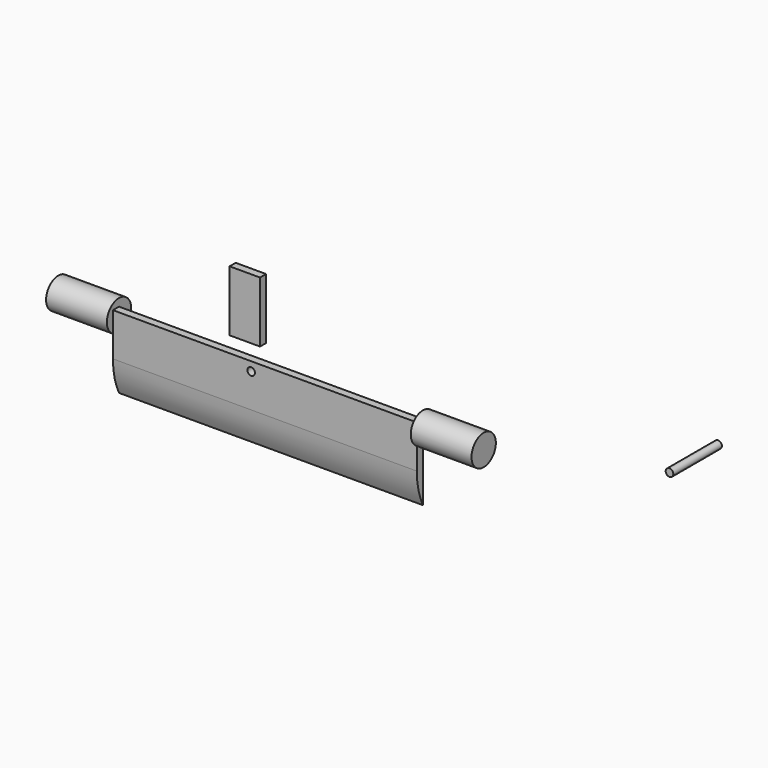
from build123d import *

# Parameters (mm, degrees)
F0_W        = 10.16
F0_H        = 2.54
F3_DEPTH    = 1.27
F4_T1_DEPTH = 78.4790082915
F5_R        = 0.635
F6_DEPTH    = 3.811
F7_DEPTH    = 10.16
F8_DEPTH    = 1.27


# Not quite as in the source:
# - a fillet or chamfer that OpenCascade refuses, or shapes differently, is made with other operations: its cross-section is extruded or revolved along the edge and cut away or added


with BuildPart() as f1:
    # F0 (on Front) → F1 (revolve)
    with BuildSketch(Plane.XZ):
        with Locations((-53.6708150854, 36.4173984443)):
            Rectangle(F0_W, F0_H)
    revolve(axis=Axis((-53.6708150854, 0, 37.6873984443), (-1, 0, 0)))


with BuildPart() as f2:
    # F0 (on Front) → F2 (revolve)
    with BuildSketch(Plane.XZ):
        with Locations((7.2891849146, 36.4173984443)):
            Rectangle(F0_W, F0_H)
    revolve(axis=Axis((7.2891849146, 0, 37.6873984443), (1, 0, 0)))


with BuildPart() as f3:
    # F0 (on Front) → F3 (new body)
    with BuildSketch(Plane.XZ):
        Polygon((-48.5908150854, 26.2573984443), (2.2091849146, 26.2573984443), (2.2091849146, 35.1473984443), (2.2091849146, 37.6873984443), (2.2091849146, 38.9573984443), (-48.5908150854, 38.9573984443), (-48.5908150854, 37.6873984443), (-48.5908150854, 35.1473984443), align=None)
    extrude(amount=F3_DEPTH)

    # F4: fillet of radius 12.7 on 1 edges, made by hand

    # F4_s2 → F4_t1 (cut)
    with BuildSketch(Plane.YZ.offset(-62.4303192311)):
        with BuildLine():
            add(Edge.make_bspline(
                [(0, 26.2573984443), (-1.27, 28.8796202825), (-1.27, 31.7932001026)],
                knots=[0, 0, 0, 1, 1, 1], degree=2, weights=[1, 1, 1]))
            Line((-1.27, 31.7932001026), (-1.524, 31.7932001026))
            Line((-1.524, 31.7932001026), (-1.524, 26.2573984443))
            Line((-1.524, 26.2573984443), (-1.27, 26.0033984443))
            ThreePointArc((-1.27, 26.0033984443), (-0.635, 26.0033984443), (-0.2286, 26.1466824112))
            Line((-0.2286, 26.1466824112), (0, 26.2573984443))
        make_face()
    extrude(amount=F4_T1_DEPTH, mode=Mode.SUBTRACT)

    # F5 (on face) → F6 (cut, through all)
    with BuildSketch(Plane.XZ.offset(1.27)):
        with Locations((-25.4863388836, 37.4436601996)):
            Circle(F5_R)
    extrude(amount=-F6_DEPTH, mode=Mode.SUBTRACT)


with BuildPart() as f7:
    # F5 (on face) → F7 (new body)
    with BuildSketch(Plane.XZ.offset(1.27)):
        with Locations((52.5741390884, 52.078012377)):
            Circle(F5_R)
    extrude(amount=F7_DEPTH)


with BuildPart() as f8:
    # F0 (on Front) → F8 (new body)
    with BuildSketch(Plane.XZ):
        Polygon((-29.0838461369, 51.7536484933), (-29.0838461369, 45.0394451618), (-29.0838461369, 41.5936484933), (-24.0038461369, 41.5936484933), (-24.0038461369, 51.7536484933), align=None)
    extrude(amount=F8_DEPTH)


solid = Compound([f1.part, f2.part, f3.part, f7.part, f8.part])
